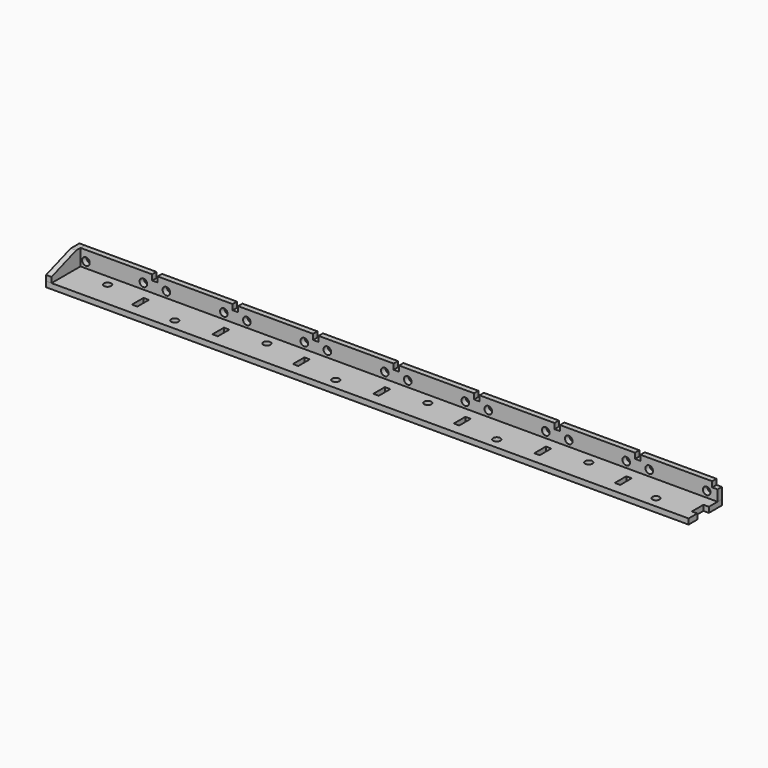
from build123d import *

# Parameters (mm, degrees)
F0_W      = 354.9
F0_H      = 12
F0_R      = 2.1
F3_DEPTH  = 3
F1_W      = 3
F1_H      = 3
F1_W_2    = 1.5
F1_W_3    = 4.4
F1_W_4    = 4.6055555556
F4_DEPTH  = 3.001
F2_W      = 354.9
F2_H      = 3
F5_DEPTH  = 23
F7_W      = 3
F7_H      = 8
F8_DEPTH  = 3.001
F9_R      = 2
F10_DEPTH = 3.001
F11_W     = 3
F11_H     = 3
F12_DEPTH = 3.001
F14_DEPTH = 3


# Not quite as in the source:
# - a feature names something its author has since deleted; it is built from what else it names


with BuildPart() as f3:
    # F0 (on Front) → F3 (new body)
    with BuildSketch(Plane.XZ):
        with Locations((177.45, 6)):
            Rectangle(F0_W, F0_H)
        with Locations((6, 6.35)):
            Circle(F0_R, mode=Mode.SUBTRACT)
        with Locations((37.75, 6.35)):
            Circle(F0_R, mode=Mode.SUBTRACT)
        with Locations((50.45, 6.35)):
            Circle(F0_R, mode=Mode.SUBTRACT)
        with Locations((82.2, 6.35)):
            Circle(F0_R, mode=Mode.SUBTRACT)
        with Locations((94.9, 6.35)):
            Circle(F0_R, mode=Mode.SUBTRACT)
        with Locations((126.65, 6.35)):
            Circle(F0_R, mode=Mode.SUBTRACT)
        with Locations((139.35, 6.35)):
            Circle(F0_R, mode=Mode.SUBTRACT)
        with Locations((171.1, 6.35)):
            Circle(F0_R, mode=Mode.SUBTRACT)
        with Locations((183.8, 6.35)):
            Circle(F0_R, mode=Mode.SUBTRACT)
        with Locations((215.55, 6.35)):
            Circle(F0_R, mode=Mode.SUBTRACT)
        with Locations((228.25, 6.35)):
            Circle(F0_R, mode=Mode.SUBTRACT)
        with Locations((260, 6.35)):
            Circle(F0_R, mode=Mode.SUBTRACT)
        with Locations((272.7, 6.35)):
            Circle(F0_R, mode=Mode.SUBTRACT)
        with Locations((304.45, 6.35)):
            Circle(F0_R, mode=Mode.SUBTRACT)
        with Locations((317.15, 6.35)):
            Circle(F0_R, mode=Mode.SUBTRACT)
        with Locations((348.9, 6.35)):
            Circle(F0_R, mode=Mode.SUBTRACT)
    extrude(amount=F3_DEPTH)

    # F1 (on face) → F4 (cut, through all)
    with BuildSketch(Plane.XZ):
        with Locations((1.5, 1.5)):
            Rectangle(F1_W, F1_H)
        with Locations((44.1, 1.5)):
            Rectangle(F1_W, F1_H)
        with Locations((353.4, 1.5)):
            Rectangle(F1_W, F1_H)
        with Locations((88.55, 1.5)):
            Rectangle(F1_W, F1_H)
        with Locations((133, 1.5)):
            Rectangle(F1_W, F1_H)
        with Locations((178.2, 1.5)):
            Rectangle(F1_W_2, F1_H)
        with Locations((222.65, 1.5)):
            Rectangle(F1_W_2, F1_H)
        with Locations((311.55, 1.5)):
            Rectangle(F1_W_2, F1_H)
        with Locations((221.15, 1.5)):
            Rectangle(F1_W_2, F1_H)
        with Locations((176.7, 1.5)):
            Rectangle(F1_W_2, F1_H)
        with Locations((266.35, 1.5)):
            Rectangle(F1_W, F1_H)
        with Locations((345.3, 1.5)):
            Rectangle(F1_W_3, F1_H)
        with Locations((336.5, 1.5)):
            Rectangle(F1_W_3, F1_H)
        with Locations((327.7, 1.5)):
            Rectangle(F1_W_3, F1_H)
        with Locations((318.9, 1.5)):
            Rectangle(F1_W_3, F1_H)
        with Locations((302.3916666667, 1.5)):
            Rectangle(F1_W_4, F1_H)
        with Locations((310.05, 1.5)):
            Rectangle(F1_W_2, F1_H)
        with Locations((293.1805555556, 1.5)):
            Rectangle(F1_W_4, F1_H)
        with Locations((283.9694444444, 1.5)):
            Rectangle(F1_W_4, F1_H)
        with Locations((274.7583333333, 1.5)):
            Rectangle(F1_W_4, F1_H)
        with Locations((257.9416666667, 1.5)):
            Rectangle(F1_W_4, F1_H)
        with Locations((248.7305555556, 1.5)):
            Rectangle(F1_W_4, F1_H)
        with Locations((239.5194444444, 1.5)):
            Rectangle(F1_W_4, F1_H)
        with Locations((230.3083333333, 1.5)):
            Rectangle(F1_W_4, F1_H)
        with Locations((213.4916666667, 1.5)):
            Rectangle(F1_W_4, F1_H)
        with Locations((204.2805555556, 1.5)):
            Rectangle(F1_W_4, F1_H)
        with Locations((195.0694444444, 1.5)):
            Rectangle(F1_W_4, F1_H)
        with Locations((185.8583333333, 1.5)):
            Rectangle(F1_W_4, F1_H)
        with Locations((169.0416666667, 1.5)):
            Rectangle(F1_W_4, F1_H)
        with Locations((159.8305555556, 1.5)):
            Rectangle(F1_W_4, F1_H)
        with Locations((150.6194444444, 1.5)):
            Rectangle(F1_W_4, F1_H)
        with Locations((141.4083333333, 1.5)):
            Rectangle(F1_W_4, F1_H)
        with Locations((124.5916666667, 1.5)):
            Rectangle(F1_W_4, F1_H)
        with Locations((115.3805555556, 1.5)):
            Rectangle(F1_W_4, F1_H)
        with Locations((106.1694444444, 1.5)):
            Rectangle(F1_W_4, F1_H)
        with Locations((96.9583333333, 1.5)):
            Rectangle(F1_W_4, F1_H)
        with Locations((80.1416666667, 1.5)):
            Rectangle(F1_W_4, F1_H)
        with Locations((70.9305555556, 1.5)):
            Rectangle(F1_W_4, F1_H)
        with Locations((61.7194444444, 1.5)):
            Rectangle(F1_W_4, F1_H)
        with Locations((52.5083333333, 1.5)):
            Rectangle(F1_W_4, F1_H)
        with Locations((36, 1.5)):
            Rectangle(F1_W_3, F1_H)
        with Locations((27.2, 1.5)):
            Rectangle(F1_W_3, F1_H)
        with Locations((9.6, 1.5)):
            Rectangle(F1_W_3, F1_H)
        with Locations((18.4, 1.5)):
            Rectangle(F1_W_3, F1_H)
    extrude(amount=F4_DEPTH, mode=Mode.SUBTRACT)


with BuildPart() as f5:
    # F2 (on Front) → F5 (new body)
    with BuildSketch(Plane.XZ):
        with Locations((177.45, 1.5)):
            Rectangle(F2_W, F2_H)
    extrude(amount=F5_DEPTH)

    # F6: cut F3
    add(f3.part, mode=Mode.SUBTRACT)

    # F7 (on face) → F8 (cut, through all)
    with BuildSketch(Plane.XY.offset(3)):
        with Locations((353.4, -13)):
            Rectangle(F7_W, F7_H)
        with Locations((221.9, -13)):
            Rectangle(F7_W, F7_H)
        with Locations((266.35, -13)):
            Rectangle(F7_W, F7_H)
        with Locations((310.8, -13)):
            Rectangle(F7_W, F7_H)
        with Locations((177.45, -13)):
            Rectangle(F7_W, F7_H)
        with Locations((133, -13)):
            Rectangle(F7_W, F7_H)
        with Locations((88.55, -13)):
            Rectangle(F7_W, F7_H)
        with Locations((44.1, -13)):
            Rectangle(F7_W, F7_H)
        with Locations((1.5, -13)):
            Rectangle(F7_W, F7_H)
    extrude(amount=-F8_DEPTH, mode=Mode.SUBTRACT)

    # F9 (on face) → F10 (cut, through all)
    with BuildSketch(Plane.XY.offset(3)):
        with Locations((332.1, -17)):
            Circle(F9_R)
        with Locations((288.575, -9)):
            Circle(F9_R)
        with Locations((244.125, -17)):
            Circle(F9_R)
        with BuildLine():
            ThreePointArc((157.225, -17), (155.225, -15), (153.225, -17))
            Line((153.225, -17), (157.225, -17))
        make_face()
        with BuildLine():
            Line((157.225, -17), (153.225, -17))
            ThreePointArc((153.225, -17), (155.225, -19), (157.225, -17))
        make_face()
        with Locations((199.675, -9)):
            Circle(F9_R)
        with Locations((66.325, -17)):
            Circle(F9_R)
        with Locations((110.775, -9)):
            Circle(F9_R)
        with Locations((22.8, -9)):
            Circle(F9_R)
    extrude(amount=-F10_DEPTH, mode=Mode.SUBTRACT)


with BuildPart() as f3_1:
    add(f3.part)

    # F11 (on face) → F12 (cut, through all)
    with BuildSketch(Plane.XZ.offset(3)):
        with Locations((1.5, 10.5)):
            Rectangle(F11_W, F11_H)
        with Locations((44.1, 10.5)):
            Rectangle(F11_W, F11_H)
        with Locations((88.55, 10.5)):
            Rectangle(F11_W, F11_H)
        with Locations((133, 10.5)):
            Rectangle(F11_W, F11_H)
        with Locations((177.45, 10.5)):
            Rectangle(F11_W, F11_H)
        with Locations((221.9, 10.5)):
            Rectangle(F11_W, F11_H)
        with Locations((266.35, 10.5)):
            Rectangle(F11_W, F11_H)
        with Locations((310.8, 10.5)):
            Rectangle(F11_W, F11_H)
        with Locations((353.4, 10.5)):
            Rectangle(F11_W, F11_H)
    extrude(amount=-F12_DEPTH, mode=Mode.SUBTRACT)


with BuildPart() as f14:
    # F13 (on face) → F14 (new body)
    with BuildSketch(Plane(origin=(0, 0, 0), x_dir=(0, -1, 0), z_dir=(-1, 0, 0))):
        Polygon((17, 3), (23, 3), (23, 6), (6, 12), (0, 12), (0, 9), (3, 9), (3, 3), (9, 3), (9, 0), (17, 0), align=None)
    extrude(amount=-F14_DEPTH)


solid = Compound([f5.part, f3_1.part, f14.part])
